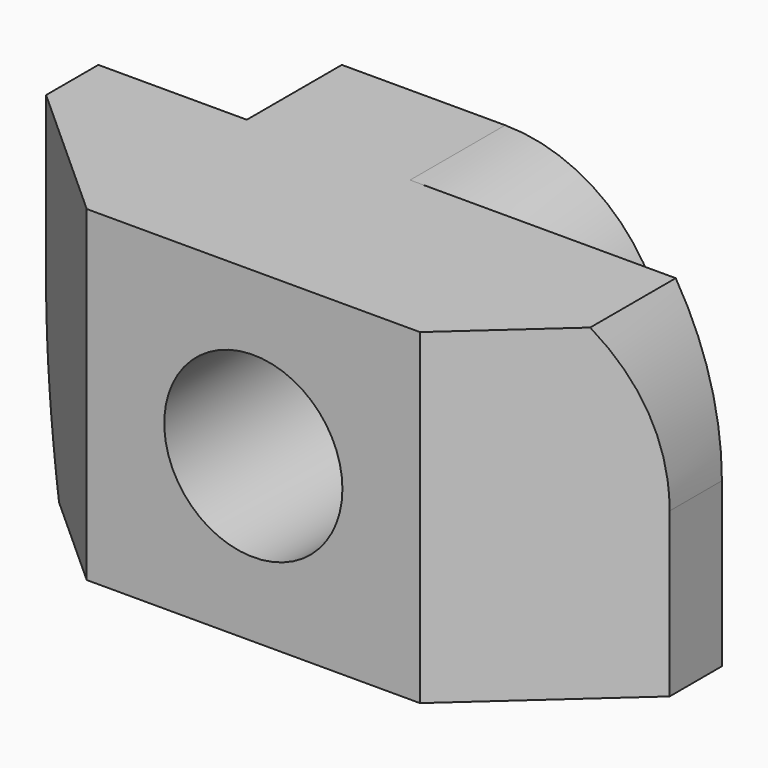
from build123d import *
from build123d import SkipClean  # not in build123d's __all__

# Parameters (mm, degrees)
F0_R     = 1.5
F1_DEPTH = 3.8
F3_DEPTH = 2
F5_DEPTH = 25
F6_W     = 5.9742073228
F6_H     = 0.5
F7_DEPTH = 25


# Not quite as in the source:
# - after a boolean that leaves OpenCascade's solid faulty, fix() repairs it


with BuildPart() as f1:
    # F0 (on Front) → F1 (new body)
    with BuildSketch(Plane.XZ):
        with BuildLine():
            Line((-4.472135955, -2.75), (4.472135955, -2.75))
            ThreePointArc((4.472135955, -2.75), (5.0517924425, -1.4289482559), (5.25, 0))
            ThreePointArc((5.25, 0), (5.0517924425, 1.4289482559), (4.472135955, 2.75))
            Line((4.472135955, 2.75), (-4.472135955, 2.75))
            ThreePointArc((-4.472135955, 2.75), (-5.0517924425, 1.4289482559), (-5.25, 0))
            ThreePointArc((-5.25, 0), (-5.0517924425, -1.4289482559), (-4.472135955, -2.75))
        make_face()
        Circle(F0_R, mode=Mode.SUBTRACT)
        with BuildLine():
            Line((-5.25, 2.75), (-5.25, 0))
            ThreePointArc((-5.25, 0), (-5.0517924425, 1.4289482559), (-4.472135955, 2.75))
            Line((-4.472135955, 2.75), (-5.25, 2.75))
        make_face()
        with BuildLine():
            Line((4.472135955, -2.75), (5.25, -2.75))
            Line((5.25, -2.75), (5.25, 0))
            ThreePointArc((5.25, 0), (5.0517924425, -1.4289482559), (4.472135955, -2.75))
        make_face()
    extrude(amount=F1_DEPTH)

    # F2 (on face) → F3 (join)
    with BuildSketch(Plane(origin=(0, 0, 0), x_dir=(-1, 0, 0), z_dir=(0, 1, 0))):
        with BuildLine():
            Line((1.5, 0), (2.75, 0))
            ThreePointArc((2.75, 0), (1.9445436483, 1.9445436483), (0, 2.75))
            ThreePointArc((0, 2.75), (-1.9445436483, 1.9445436483), (-2.75, 0))
            Line((-2.75, 0), (-1.5, 0))
            ThreePointArc((-1.5, 0), (0, 1.5), (1.5, 0))
        make_face()
        with BuildLine():
            ThreePointArc((0, -2.75), (1.9445436483, -1.9445436483), (2.75, 0))
            Line((2.75, 0), (1.5, 0))
            ThreePointArc((1.5, 0), (0, -1.5), (-1.5, 0))
            Line((-1.5, 0), (-2.75, 0))
            ThreePointArc((-2.75, 0), (-1.9445436483, -1.9445436483), (0, -2.75))
        make_face()
        with BuildLine():
            ThreePointArc((0, 2.75), (1.9445436483, 1.9445436483), (2.75, 0))
            Line((2.75, 0), (2.75, 2.75))
            Line((2.75, 2.75), (0, 2.75))
        make_face()
        with BuildLine():
            Line((-2.75, -2.75), (0, -2.75))
            ThreePointArc((0, -2.75), (-1.9445436483, -1.9445436483), (-2.75, 0))
            Line((-2.75, 0), (-2.75, -2.75))
        make_face()
    with SkipClean():  # cleaning this boolean's faces spoils the solid; the shape is the same uncleaned
        extrude(amount=F3_DEPTH)

    # F4 (on face) → F5 (cut)
    with BuildSketch(Plane.XY.offset(2.75)):
        Polygon((-5.25, -1.1), (-5.25, -3.8), (-2.25, -3.8), align=None)
        Polygon((2.25, -3.8), (5.25, -3.8), (5.25, -1.1), align=None)
    extrude(amount=-F5_DEPTH, mode=Mode.SUBTRACT)

    add(f1.part.fix(), mode=Mode.REPLACE)

    # F6 (on face) → F7 (cut)
    with BuildSketch(Plane.XY.offset(2.75)):
        with Locations((-0.0664879346, -3.55)):
            Rectangle(F6_W, F6_H)
    extrude(amount=-F7_DEPTH, mode=Mode.SUBTRACT)


solid = f1.part
